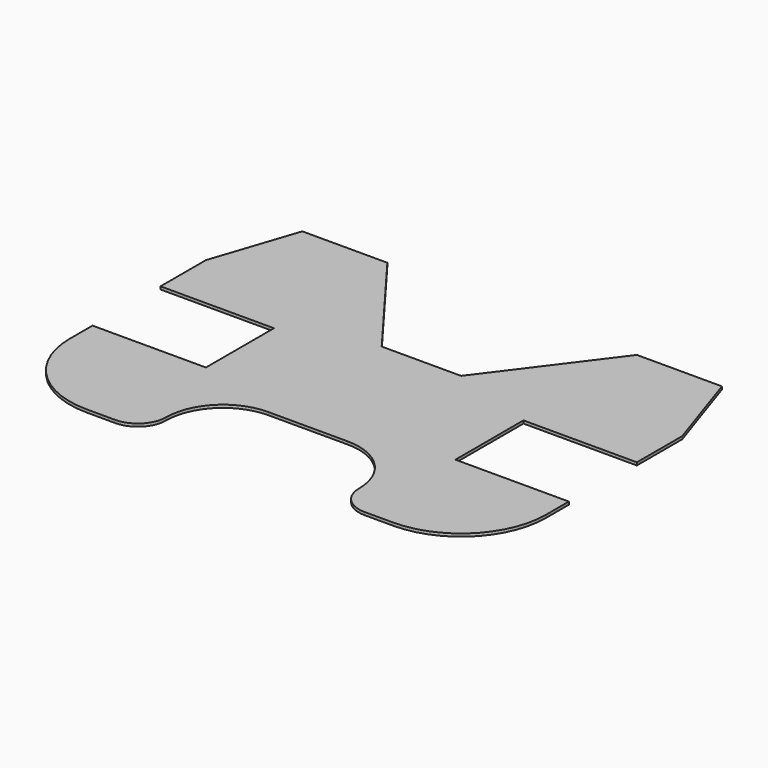
from build123d import *

# Parameters (mm, degrees)
F0_W      = 440
F0_H      = 250
F1_DEPTH  = 5
F2_W      = 250
F2_H      = 200
F2_W_2    = 350
F2_H_2    = 250
F3_DEPTH  = 5
F4_R      = 150
F5_R      = 100
F6_R      = 49.99999
F7_SIZE2  = 150
F7_SIZE   = 50
F8_SIZE2  = 50
F8_SIZE   = 150
F10_DEPTH = 25


# Not quite as in the source:
# - a fillet or chamfer is up to 0.001 mm smaller than in the source, because OpenCascade refuses the exact size


with BuildPart() as f1:
    # F0 (on Top) → F1 (new body)
    with BuildSketch(Plane.XY):
        Rectangle(F0_W, F0_H)
    extrude(amount=F1_DEPTH)

    # F2 (on face) → F3 (join)
    with BuildSketch(Plane(origin=(0, 0, 0), x_dir=(1, 0, 0), z_dir=(0, 0, -1))):
        with Locations((-295, 175)):
            Rectangle(F2_W, F2_H)
        with Locations((295, 175)):
            Rectangle(F2_W, F2_H)
        with Locations((-245, -200)):
            Rectangle(F2_W_2, F2_H_2)
        with Locations((245, -200)):
            Rectangle(F2_W_2, F2_H_2)
    extrude(amount=-F3_DEPTH)

    # F4
    f4_edges = [f1.edges().sort_by_distance(p)[0] for p in [
        (-420, -275, 2.5),
        (420, -275, 2.5),
    ]]
    fillet(f4_edges, radius=F4_R)

    # F5
    f5_edges = [f1.edges().sort_by_distance(p)[0] for p in [
        (170, -125, 2.5),
        (-170, -125, 2.5),
    ]]
    fillet(f5_edges, radius=F5_R)

    # F6 (radius 50 in the source; OpenCascade refuses exactly that, so slightly less here)
    f6_edges = [f1.edges().sort_by_distance(p)[0] for p in [
        (-170, -275, 2.5),
        (170, -275, 2.5),
    ]]
    fillet(f6_edges, radius=F6_R)

    # F7
    f7_edges = [f1.edges().sort_by_distance(p)[0] for p in [
        (420, 325, 2.5),
    ]]
    f7_side = f1.faces().sort_by_distance((245, 325, 2.5))[0]
    chamfer(f7_edges, length=F7_SIZE, length2=F7_SIZE2, reference=f7_side)

    # F8
    f8_edges = [f1.edges().sort_by_distance(p)[0] for p in [
        (-420, 325, 2.5),
    ]]
    f8_side = f1.faces().sort_by_distance((-420, 200, 2.5))[0]
    chamfer(f8_edges, length=F8_SIZE, length2=F8_SIZE2, reference=f8_side)

    # F9 (on face) → F10 (cut)
    with BuildSketch(Plane.XY.offset(5)):
        Polygon((-220, 325), (-70, 125), (-70, 325), align=None)
        Polygon((70, 325), (70, 125), (220, 325), align=None)
    extrude(amount=-F10_DEPTH, mode=Mode.SUBTRACT)


solid = f1.part
